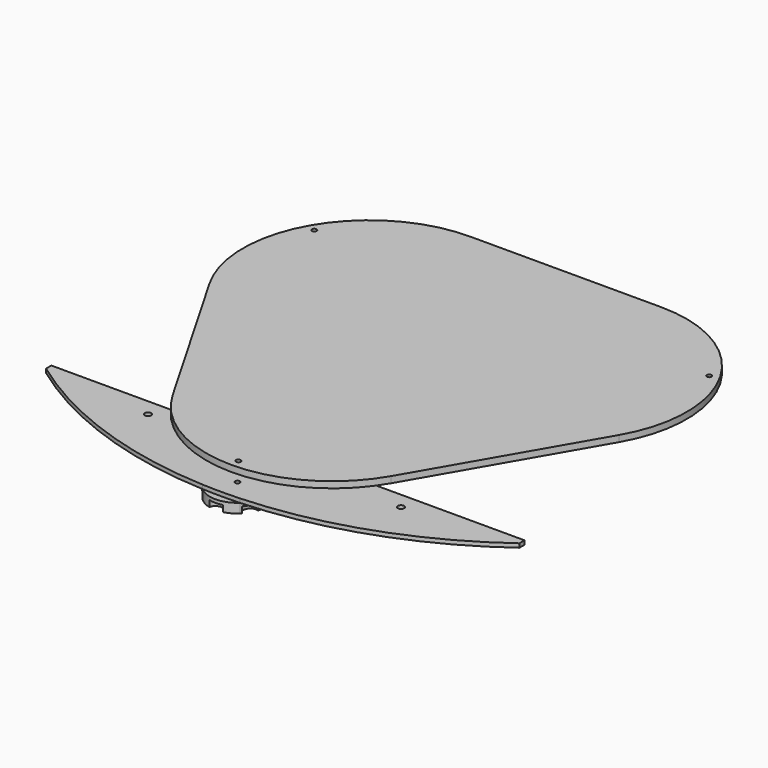
from build123d import *

# Parameters (mm, degrees)
F0_R     = 2
F0_R_2   = 1.5
F1_DEPTH = 2.5
F2_DEPTH = 6
F3_R     = 1.5
F4_DEPTH = 4
F6_R     = 1.5
F7_DEPTH = 4


with BuildPart() as f1:
    # F0 (on Top) → F1 (new body)
    with BuildSketch(Plane.XY):
        with BuildLine():
            Line((89.1861994347, -28.6264261603), (-210.8138005653, -28.6264261603))
            Line((-210.8138005653, -28.6264261603), (-210.8138005653, -32.8214745699))
            ThreePointArc((-210.8138005653, -32.8214745699), (-145.3037250806, -67.3786400235), (-72.6072331904, -81.5556545564))
            ThreePointArc((-72.6072331904, -81.5556545564), (-67.8800912847, -52.6165062521), (-43.3138005653, -68.6264261603))
            ThreePointArc((-43.3138005653, -68.6264261603), (-44.8017830034, -75.6879623669), (-49.012691262, -81.548648075))
            ThreePointArc((-49.012691262, -81.548648075), (23.6878126625, -67.3240641933), (89.1861994347, -32.7167905686))
            Line((89.1861994347, -32.7167905686), (89.1861994347, -28.6264261603))
        make_face()
        with Locations((-140.8487898659, -39.5672686244)):
            Circle(F0_R, mode=Mode.SUBTRACT)
        with Locations((19.1502383088, -39.0096099949)):
            Circle(F0_R, mode=Mode.SUBTRACT)
        with BuildLine():
            ThreePointArc((-43.3138005653, -68.6264261603), (-67.8800912847, -52.6165062521), (-72.6072331904, -81.5556545564))
            ThreePointArc((-72.6072331904, -81.5556545564), (-60.8098807792, -81.8264265401), (-49.012691262, -81.548648075))
            ThreePointArc((-49.012691262, -81.548648075), (-44.8017830034, -75.6879623669), (-43.3138005653, -68.6264261603))
        make_face()
        with Locations((-60.8138005653, -68.6264261603)):
            Circle(F0_R_2, mode=Mode.SUBTRACT)
    extrude(amount=F1_DEPTH)


with BuildPart() as f2:
    # F0 (on Top) → F2 (new body)
    with BuildSketch(Plane.XY):
        with BuildLine():
            ThreePointArc((-43.3138005653, -68.6264261603), (-67.8800912847, -52.6165062521), (-72.6072331904, -81.5556545564))
            ThreePointArc((-72.6072331904, -81.5556545564), (-60.8098807792, -81.8264265401), (-49.012691262, -81.548648075))
            ThreePointArc((-49.012691262, -81.548648075), (-44.8017830034, -75.6879623669), (-43.3138005653, -68.6264261603))
        make_face()
        with Locations((-60.8138005653, -68.6264261603)):
            Circle(F0_R_2, mode=Mode.SUBTRACT)
        with BuildLine():
            ThreePointArc((-49.012691262, -81.548648075), (-60.8098807792, -81.8264265401), (-72.6072331904, -81.5556545564))
            ThreePointArc((-72.6072331904, -81.5556545564), (-60.8086038796, -86.1264253887), (-49.012691262, -81.548648075))
        make_face()
    extrude(amount=-F2_DEPTH)

    # F6 (on face) → F7 (cut)
    with BuildSketch(Plane(origin=(0, 0, -6), x_dir=(1, 0, 0), z_dir=(0, 0, -1))):
        Polygon((-63.5638005653, 70.2141394006), (-63.5638005653, 67.0387129201), (-60.8138005653, 65.4509996798), (-58.0638005653, 67.0387129201), (-58.0638005653, 70.2141394006), (-60.8138005653, 71.8018526409), align=None)
        with Locations((-60.8138005653, 68.6264261603)):
            Circle(F6_R, mode=Mode.SUBTRACT)
        with BuildLine():
            ThreePointArc((-56.5545095884, 85.6001835633), (-60.8138005653, 86.1264261603), (-65.0730915423, 85.6001835633))
            ThreePointArc((-65.0730915423, 85.6001835633), (-60.8138005653, 81.8347492273), (-56.5545095884, 85.6001835633))
        make_face()
        with BuildLine():
            ThreePointArc((-77.6431511624, 73.4246506736), (-75.9692451316, 77.3764261603), (-73.3838601855, 80.80195905))
            ThreePointArc((-73.3838601855, 80.80195905), (-79.6859463804, 79.5222646268), (-77.6431511624, 73.4246506736))
        make_face()
        with BuildLine():
            ThreePointArc((-71.6775681985, 77.3764261603), (-72.1277527241, 79.2899117183), (-73.3838601855, 80.80195905))
            ThreePointArc((-73.3838601855, 80.80195905), (-75.9692451316, 77.3764261603), (-77.6431511624, 73.4246506736))
            ThreePointArc((-77.6431511624, 73.4246506736), (-73.5991578972, 73.7985528536), (-71.6775681985, 77.3764261603))
        make_face()
        with BuildLine():
            ThreePointArc((-43.9844499682, 73.4246506736), (-45.6583559991, 77.3764261603), (-48.2437409452, 80.80195905))
            ThreePointArc((-48.2437409452, 80.80195905), (-49.375057248, 75.2305876938), (-43.9844499682, 73.4246506736))
        make_face()
        with BuildLine():
            ThreePointArc((-41.3666790661, 77.3764261603), (-43.7448704411, 81.2179185678), (-48.2437409452, 80.80195905))
            ThreePointArc((-48.2437409452, 80.80195905), (-45.6583559991, 77.3764261603), (-43.9844499682, 73.4246506736))
            ThreePointArc((-43.9844499682, 73.4246506736), (-42.0804826924, 75.006338926), (-41.3666790661, 77.3764261603))
        make_face()
        with BuildLine():
            ThreePointArc((-71.6775681985, 59.8764261603), (-73.5991578972, 63.4542994671), (-77.6431511624, 63.828201647))
            ThreePointArc((-77.6431511624, 63.828201647), (-75.9692451316, 59.8764261603), (-73.3838601855, 56.4508932707))
            ThreePointArc((-73.3838601855, 56.4508932707), (-72.1277527241, 57.9629406023), (-71.6775681985, 59.8764261603))
        make_face()
        with BuildLine():
            ThreePointArc((-48.2437409452, 56.4508932707), (-45.6583559991, 59.8764261603), (-43.9844499682, 63.828201647))
            ThreePointArc((-43.9844499682, 63.828201647), (-49.375057248, 62.0222646268), (-48.2437409452, 56.4508932707))
        make_face()
        with BuildLine():
            ThreePointArc((-56.5545095884, 51.6526687574), (-60.8138005653, 55.4181030934), (-65.0730915423, 51.6526687574))
            ThreePointArc((-65.0730915423, 51.6526687574), (-60.8138005653, 51.1264261603), (-56.5545095884, 51.6526687574))
        make_face()
    extrude(amount=-F7_DEPTH, mode=Mode.SUBTRACT)


with BuildPart() as f4:
    # F3 (on Top) → F4 (new body)
    with BuildSketch(Plane.XY):
        with BuildLine():
            Line((-60.8887979234, 191.6074208131), (-121.5105761883, 191.6074208131))
            ThreePointArc((-121.5105761883, 191.6074208131), (-190.7926084911, 151.6074208131), (-190.7926084911, 71.6074208131))
            Line((-190.7926084911, 71.6074208131), (-160.4817212046, 19.1074240104))
            Line((-160.4817212046, 19.1074240104), (-130.1708302261, -33.3925791869))
            ThreePointArc((-130.1708302261, -33.3925791869), (-60.8887979234, -73.3925791869), (8.3932343794, -33.3925791869))
            Line((8.3932343794, -33.3925791869), (38.7041238567, 19.1074214104))
            Line((38.7041238567, 19.1074214104), (69.0150126443, 71.6074208131))
            ThreePointArc((69.0150126443, 71.6074208131), (69.0150126443, 151.6074208131), (-0.2670196585, 191.6074208131))
            Line((-0.2670196585, 191.6074208131), (-60.8887979234, 191.6074208131))
        make_face()
        with Locations((-60.8190901713, -67.8928421625)):
            Circle(F3_R, mode=Mode.SUBTRACT)
        with Locations((-186.0645503898, 148.7971836167)):
            Circle(F3_R, mode=Mode.SUBTRACT)
        with Locations((64.2172467909, 148.917920985)):
            Circle(F3_R, mode=Mode.SUBTRACT)
    extrude(amount=F4_DEPTH)


with BuildPart() as f4_1:
    # F5: moved
    add(f4.part.moved(Location((0, 0, 10))))


solid = Compound([f1.part, f2.part, f4_1.part])
